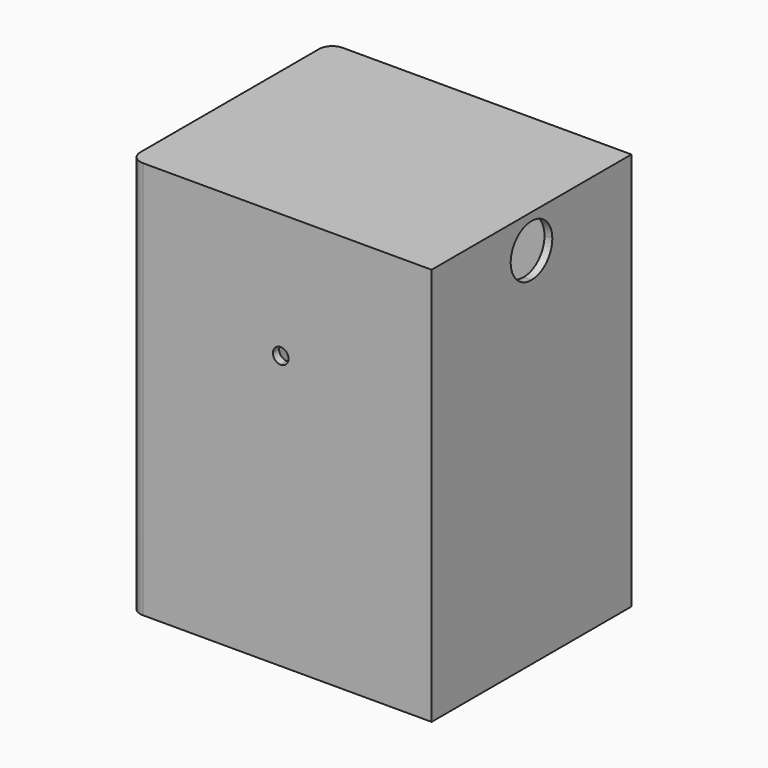
from build123d import *

# Parameters (mm, degrees)
F0_W          = 110
F0_H          = 90
F1_DEPTH      = 75
F2_T          = 3
F4_DEPTH      = 25.4
F5_W          = 3
F5_H          = 60
F6_DEPTH      = 110
F8_DEPTH      = 76
F8_DEPTH_BACK = 88
F9_R          = 5


with BuildPart() as f1:
    # F0 (on Top) → F1 (new body, symmetric)
    with BuildSketch(Plane.XY):
        Rectangle(F0_W, F0_H)
    extrude(amount=F1_DEPTH, both=True)

    # F2
    f2_openings = [f1.faces().sort_by_distance(p)[0] for p in [
        (0, 0, -75),
    ]]
    offset(amount=F2_T, openings=f2_openings, kind=Kind.INTERSECTION)

    # F3 (on face) → F4 (cut)
    with BuildSketch(Plane.YZ.offset(58)):
        with BuildLine():
            Line((0, 55), (0, 75))
            ThreePointArc((0, 75), (-7.0710678119, 72.0710678119), (-10, 65))
            ThreePointArc((-10, 65), (-7.0710678119, 57.9289321881), (0, 55))
        make_face()
        with BuildLine():
            ThreePointArc((10, 65), (7.0710678119, 72.0710678119), (0, 75))
            Line((0, 75), (0, 55))
            ThreePointArc((0, 55), (7.0710678119, 57.9289321881), (10, 65))
        make_face()
    extrude(amount=-F4_DEPTH, mode=Mode.SUBTRACT)

    # F5 (on face) → F6 (join)
    with BuildSketch(Plane(origin=(55, 0, 0), x_dir=(0, -1, 0), z_dir=(-1, 0, 0))):
        with Locations((-23.5, 48)):
            Rectangle(F5_W, F5_H)
    extrude(amount=F6_DEPTH)

    # F7 (on face) → F8 (cut, two sides)
    with BuildSketch(Plane(origin=(0, -45, 0), x_dir=(-1, 0, 0), z_dir=(0, 1, 0))) as f8_sk:
        with BuildLine():
            ThreePointArc((3, 30), (-2.1213203436, 32.1213203436), (0, 27))
            ThreePointArc((0, 27), (2.1213203436, 27.8786796564), (3, 30))
        make_face()
    extrude(amount=-F8_DEPTH, mode=Mode.SUBTRACT)
    extrude(f8_sk.sketch, amount=F8_DEPTH_BACK, mode=Mode.SUBTRACT)

    # F9
    f9_edges = [f1.edges().sort_by_distance(p)[0] for p in [
        (-58, 48, 1.5),
        (-58, -48, 1.5),
    ]]
    fillet(f9_edges, radius=F9_R)


solid = f1.part
